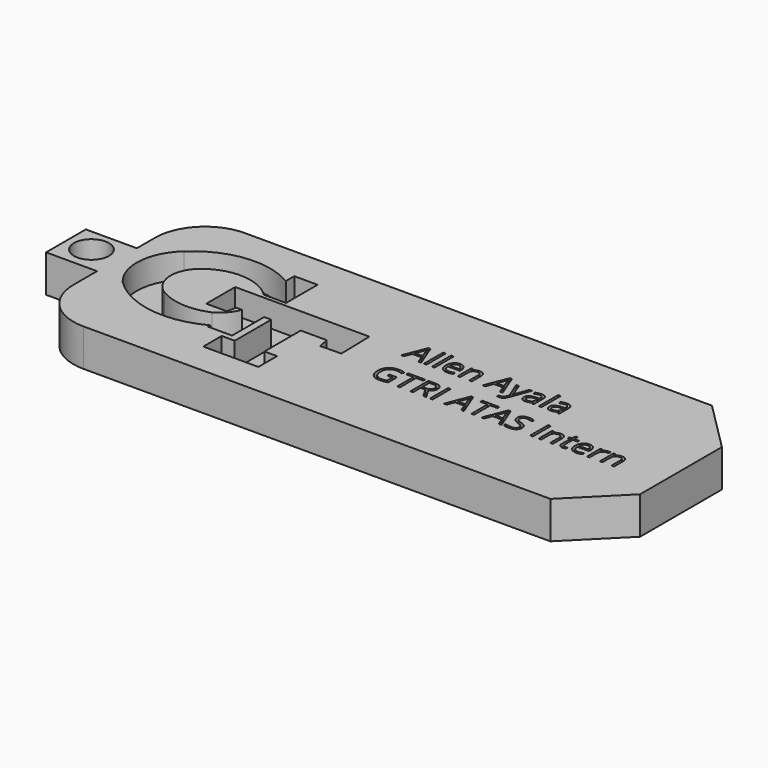
from build123d import *

# Parameters (mm, degrees)
F0_W         = 57.7379241586
F0_H         = 20.5774586648
F1_DEPTH     = 3.81
F3_DEPTH     = 2.54
F4_SIZE      = 5.08
F5_R         = 5.08
F7_W         = 5.1950379275
F7_H         = 5.0614601932
F7_R         = 1.7778769648
F8_DEPTH     = 3.81
F6_TEXT_SIZE = 3.2239255895
F9_DEPTH     = 2.54


# Not quite as in the source:
# - Text() gives the source's letters only with a copy of the font that has no kerning and outlines rounded to 1/6400 em; it was checked with that copy


with BuildPart() as f1:
    # F0 (on Top) → F1 (new body)
    with BuildSketch(Plane.XY):
        with Locations((28.8689620793, -10.2887293324)):
            Rectangle(F0_W, F0_H)
    extrude(amount=F1_DEPTH)

    # F2 (on face) → F3 (cut)
    with BuildSketch(Plane.XY.offset(3.81)):
        with BuildLine():
            Line((12.8974812105, -7.3591447435), (15.1601610705, -7.3591447435))
            Line((15.1601610705, -7.3591447435), (15.1601610705, -3.3439667895))
            Line((15.1601610705, -3.3439667895), (12.7856582403, -3.3439667895))
            Line((12.7856582403, -3.3439667895), (12.7856582403, -4.4220839627))
            ThreePointArc((12.7856582403, -4.4220839627), (7.856740139, -3.3537818035), (3.2829619013, -5.4788831621))
            ThreePointArc((3.2829619013, -5.4788831621), (1.5474593957, -8.9777290168), (2.7775403578, -12.6845864579))
            ThreePointArc((2.7775403578, -12.6845864579), (7.5959648457, -15.0620973533), (12.8836566582, -14.1081120819))
            Line((12.8836566582, -14.1081120819), (12.8836566582, -14.4250039011))
            Line((12.8836566582, -14.4250039011), (15.3151787817, -14.4250039011))
            Line((15.3151787817, -14.4250039011), (15.3151787817, -10.3389974684))
            Line((15.3151787817, -10.3389974684), (16.0354524851, -10.3389974684))
            Line((16.0354524851, -10.3389974684), (16.0354524851, -14.9867003784))
            Line((16.0354524851, -14.9867003784), (14.7102316841, -14.9867003784))
            Line((14.7102316841, -14.9867003784), (14.7102316841, -17.3347964883))
            Line((14.7102316841, -17.3347964883), (20.3224848956, -17.3347964883))
            Line((20.3224848956, -17.3347964883), (20.3224848956, -14.9499522522))
            Line((20.3224848956, -14.9499522522), (19.0375037491, -14.9499522522))
            Line((19.0375037491, -14.9499522522), (19.0375037491, -10.3389974684))
            Line((19.0375037491, -10.3389974684), (21.6899253428, -10.3389974684))
            Line((21.6899253428, -10.3389974684), (21.9017147283, -11.4583319441))
            Line((21.9017147283, -11.4583319441), (24.0391939878, -11.4109460264))
            Line((24.0391939878, -11.4109460264), (23.9578913897, -7.7435565181))
            Line((23.9578913897, -7.7435565181), (10.283104144, -7.7435565181))
            Line((10.283104144, -7.7435565181), (10.283104144, -11.4171858877))
            Line((10.283104144, -11.4171858877), (12.3737175018, -11.4171858877))
            Line((12.3737175018, -11.4171858877), (12.573351787, -10.4606067762))
            Line((12.573351787, -10.4606067762), (13.1652252749, -10.4606067762))
            ThreePointArc((13.1652252749, -10.4606067762), (12.529641711, -11.5224533623), (11.571678333, -12.3059013858))
            ThreePointArc((11.571678333, -12.3059013858), (9.0107548868, -12.7440957043), (6.519855, -12.0053393766))
            ThreePointArc((6.519855, -12.0053393766), (5.0359724705, -9.4735014115), (6.3747153617, -6.8620117381))
            ThreePointArc((6.3747153617, -6.8620117381), (9.7268655751, -5.919641879), (12.8974812105, -7.3591447435))
        make_face()
    extrude(amount=-F3_DEPTH, mode=Mode.SUBTRACT)

    # F4
    f4_edges = [f1.edges().sort_by_distance(p)[0] for p in [
        (57.737924, -20.577459, 1.905),
        (57.737924, 0, 1.905),
    ]]
    chamfer(f4_edges, length=F4_SIZE)

    # F5
    f5_edges = [f1.edges().sort_by_distance(p)[0] for p in [
        (0, -20.577459, 1.905),
        (0, 0, 1.905),
    ]]
    fillet(f5_edges, radius=F5_R)

    # F7 (on Top) → F8 (join)
    with BuildSketch(Plane.XY):
        with Locations((-2.5975189637, -9.9404819775)):
            Rectangle(F7_W, F7_H)
        with Locations((-2.6798227336, -9.8334047943)):
            Circle(F7_R, mode=Mode.SUBTRACT)
    extrude(amount=F8_DEPTH)

    # F6 (on face) → F9 (cut)
    with BuildSketch(Plane.XY.offset(3.81)):
        with Locations((27.94, -8.6712264244)):
            Text('Allen Ayala', F6_TEXT_SIZE, font='Open Sans', text_align=(TextAlign.LEFT, TextAlign.BOTTOM))
        with Locations((27.94, -13.0557652262)):
            Text('GTRI ATAS Intern', F6_TEXT_SIZE, font='Open Sans', text_align=(TextAlign.LEFT, TextAlign.BOTTOM))
    extrude(amount=-F9_DEPTH, mode=Mode.SUBTRACT)


solid = f1.part
